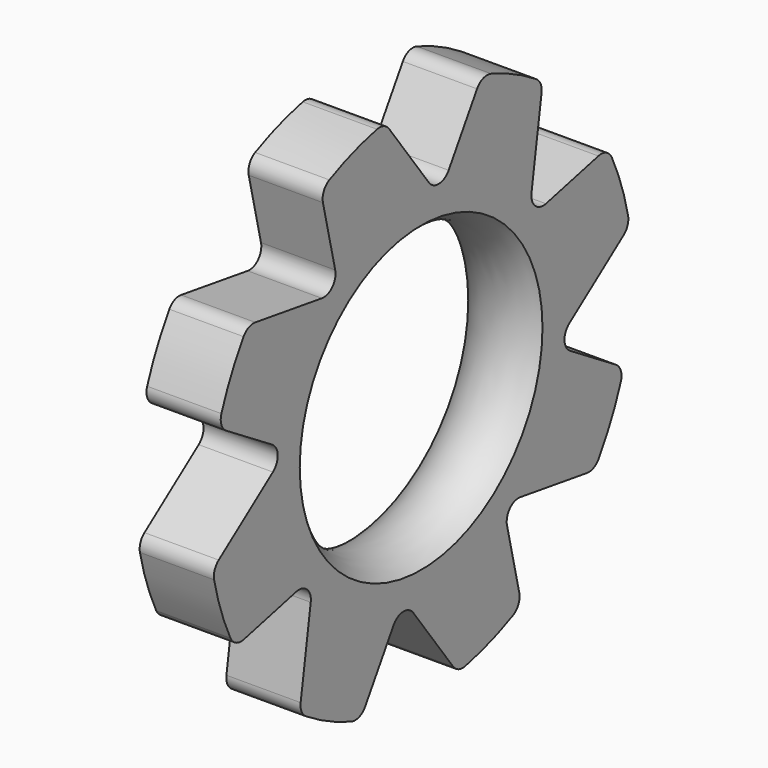
from build123d import *

# Parameters (mm, degrees)
F4_DEPTH = 60
F5_R     = 5


# Not quite as in the source:
# - a feature names something its author has since deleted; it is built from what else it names


with BuildPart() as f1:
    # F0 (on Top) → F1 (revolve)
    with BuildSketch(Plane.XY):
        with BuildLine():
            Line((-12.5, 89.1), (-12.5, 51.1))
            ThreePointArc((-12.5, 51.1), (0, 46.135443521), (12.5, 51.1))
            Line((12.5, 51.1), (12.5, 89.1))
            Line((12.5, 89.1), (-12.5, 89.1))
        make_face()
    revolve(axis=Axis((4.8881422824, 0, 0), (1, 0, 0)))

    # F3 (on offset) → F4 (cut)
    with BuildSketch(Plane.YZ.offset(15)):
        Polygon((43.1796096184, -82.538823422), (80.155778704, -52.2855824361), (34.4793311693, -45.3649125185), align=None)
        Polygon((-27.8311669827, -88.896356523), (19.707204774, -93.6501845717), (-7.6972683892, -56.4584061503), align=None)
        Polygon((-82.538823422, -43.1796096184), (-52.2855824361, -80.155778704), (-45.3649125185, -34.4793311693), align=None)
        Polygon((-56.4584061503, 7.6972683892), (-88.896356523, 27.8311669827), (-93.6501845717, -19.707204774), align=None)
        Polygon((-43.1796096184, 82.538823422), (-80.155778704, 52.2855824361), (-34.4793311693, 45.3649125185), align=None)
        Polygon((27.8311669827, 88.896356523), (-19.707204774, 93.6501845717), (7.6972683892, 56.4584061503), align=None)
        Polygon((82.538823422, 43.1796096184), (52.2855824361, 80.155778704), (45.3649125185, 34.4793311693), align=None)
        Polygon((88.896356523, -27.8311669827), (93.6501845717, 19.707204774), (56.4584061503, -7.6972683892), align=None)
    extrude(amount=-F4_DEPTH, mode=Mode.SUBTRACT)

    # F5
    f5_edges = [f1.edges().sort_by_distance(p)[0] for p in [
        (0, 87.764267, 15.370212),
        (0, 85.336625, -25.621679),
        (0, 72.92709, -51.190327),
        (0, 78.459369, 42.224844),
        (0, 51.190327, 72.92709),
        (0, 42.224844, -78.459369),
        (0, 15.370212, -87.764267),
        (0, 34.479331, -45.364913),
        (0, 56.458406, -7.697268),
        (0, 45.364913, 34.479331),
        (0, 25.621679, 85.336625),
        (0, 7.697268, 56.458406),
        (0, -15.370212, 87.764267),
        (0, -42.224844, 78.459369),
        (0, -34.479331, 45.364913),
        (0, -72.92709, 51.190327),
        (0, -85.336625, 25.621679),
        (0, -56.458406, 7.697268),
        (0, -87.764267, -15.370212),
        (0, -78.459369, -42.224844),
        (0, -45.364913, -34.479331),
        (0, -51.190327, -72.92709),
        (0, -25.621679, -85.336625),
        (0, -7.697268, -56.458406),
    ]]
    fillet(f5_edges, radius=F5_R)


solid = f1.part
